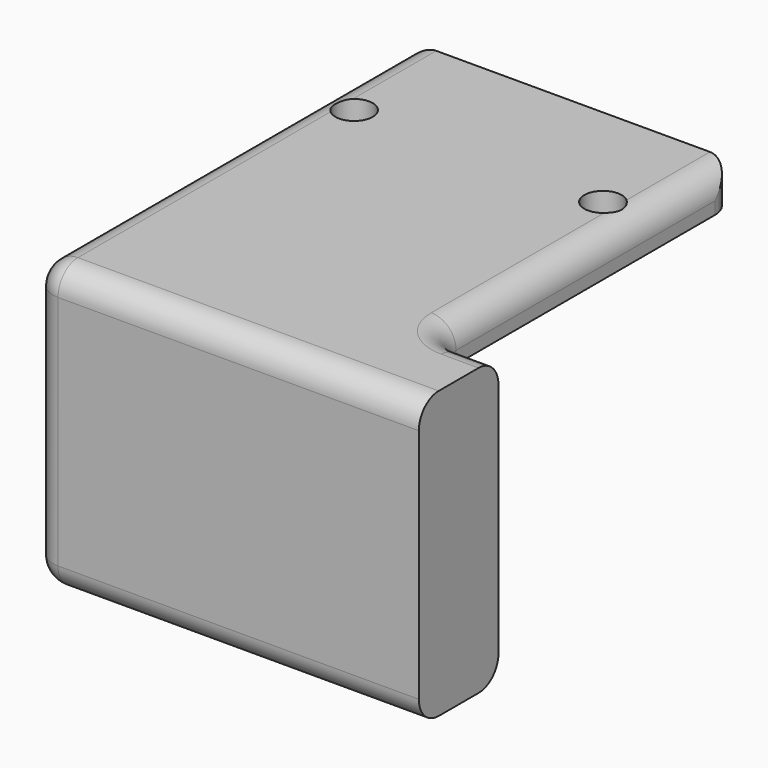
from build123d import *

# Parameters (mm, degrees)
F0_W         = 26
F0_H         = 38
F0_R         = 1.5
F1_DEPTH     = 3
F2_W         = 26
F2_H         = 8
F3_DEPTH     = 20
F5_DEPTH     = 5
F6_T1_DEPTH  = 3
F6_T3_DEPTH  = 18
F6_T5_DEPTH  = 19
F6_T7_DEPTH  = 13
F6_T9_DEPTH  = 41
F6_T11_DEPTH = 33
F6_T13_DEPTH = 34
F6_T15_DEPTH = 4
F6_T17_DEPTH = 8
F6_S21_W     = 2.04
F6_S21_H     = 2.04
F6_T22_DEPTH = 2.04
F6_S27_W     = 2.04
F6_S27_H     = 2.04
F6_T28_DEPTH = 2.04
F6_S33_W     = 2.04
F6_S33_H     = 2.04
F6_T34_DEPTH = 2.04
F6_T38_ANGLE = 90


# Not quite as in the source:
# - a fillet or chamfer that OpenCascade refuses, or shapes differently, is made with other operations: its cross-section is extruded or revolved along the edge and cut away or added


with BuildPart() as f1:
    # F0 (on Top) → F1 (new body)
    with BuildSketch(Plane.XY):
        Rectangle(F0_W, F0_H)
        with Locations((-10, 9.5)):
            Circle(F0_R, mode=Mode.SUBTRACT)
        with Locations((10, 9.5)):
            Circle(F0_R, mode=Mode.SUBTRACT)
    extrude(amount=F1_DEPTH)

    # F2 (on face) → F3 (join)
    with BuildSketch(Plane(origin=(0, 0, 0), x_dir=(1, 0, 0), z_dir=(0, 0, -1))):
        with Locations((0, 15)):
            Rectangle(F2_W, F2_H)
    extrude(amount=F3_DEPTH)

    # F4 (on face) → F5 (join)
    with BuildSketch(Plane.YZ.offset(13)):
        Polygon((-11, -20), (-11, 0), (-11, 3), (-19, 3), (-19, -20), align=None)
    extrude(amount=F5_DEPTH)

    # F6: fillet of radius 2 on 12 edges, made by hand

    # F6_s2 → F6_t1 (join)
    with BuildSketch(Plane.XY):
        with BuildLine():
            ThreePointArc((15, -11), (13.5857864376, -10.4142135624), (13, -9))
            Line((13, -9), (13, -11))
            Line((13, -11), (15, -11))
        make_face()
    extrude(amount=F6_T1_DEPTH)

    # F6_s4 → F6_t3 (cut)
    with BuildSketch(Plane.XY.offset(-18)):
        with BuildLine():
            ThreePointArc((-11, -11), (-12.4142135624, -11.5857864376), (-13, -13))
            Line((-13, -13), (-13, -11))
            Line((-13, -11), (-11, -11))
        make_face()
    extrude(amount=F6_T3_DEPTH, mode=Mode.SUBTRACT)

    # F6_s6 → F6_t5 (cut)
    with BuildSketch(Plane.XY.offset(-18)):
        with BuildLine():
            ThreePointArc((-11, -19), (-12.4142135624, -18.4142135624), (-13, -17))
            Line((-13, -17), (-13, -19))
            Line((-13, -19), (-11, -19))
        make_face()
    extrude(amount=F6_T5_DEPTH, mode=Mode.SUBTRACT)

    # F6_s8 → F6_t7 (cut)
    with BuildSketch(Plane.XY.offset(-5)):
        with BuildLine():
            ThreePointArc((13, 17), (12.4142135624, 18.4142135624), (11, 19))
            Line((11, 19), (13, 19))
            Line((13, 19), (13, 17))
        make_face()
        with BuildLine():
            ThreePointArc((-11, 19), (-12.4142135624, 18.4142135624), (-13, 17))
            Line((-13, 17), (-13, 19))
            Line((-13, 19), (-11, 19))
        make_face()
    extrude(amount=F6_T7_DEPTH, mode=Mode.SUBTRACT)

    # F6_s10 → F6_t9 (cut)
    with BuildSketch(Plane.XZ.offset(-24)):
        with BuildLine():
            ThreePointArc((-11, 3), (-12.4142135624, 2.4142135624), (-13, 1))
            Line((-13, 1), (-13, 3))
            Line((-13, 3), (-11, 3))
        make_face()
    extrude(amount=F6_T9_DEPTH, mode=Mode.SUBTRACT)

    # F6_s12 → F6_t11 (cut)
    with BuildSketch(Plane.XZ.offset(-24)):
        with BuildLine():
            ThreePointArc((13, 1), (12.4142135624, 2.4142135624), (11, 3))
            Line((11, 3), (13, 3))
            Line((13, 3), (13, 1))
        make_face()
    extrude(amount=F6_T11_DEPTH, mode=Mode.SUBTRACT)

    # F6_s14 → F6_t13 (cut)
    with BuildSketch(Plane.YZ.offset(-11)):
        with BuildLine():
            ThreePointArc((-13, -20), (-11.5857864376, -19.4142135624), (-11, -18))
            Line((-11, -18), (-11, -20))
            Line((-11, -20), (-13, -20))
        make_face()
        with BuildLine():
            ThreePointArc((-19, -18), (-18.4142135624, -19.4142135624), (-17, -20))
            Line((-17, -20), (-19, -20))
            Line((-19, -20), (-19, -18))
        make_face()
        with BuildLine():
            ThreePointArc((-19, 1), (-18.4142135624, 2.4142135624), (-17, 3))
            Line((-17, 3), (-19, 3))
            Line((-19, 3), (-19, 1))
        make_face()
    extrude(amount=F6_T13_DEPTH, mode=Mode.SUBTRACT)

    # F6_s16 → F6_t15 (cut)
    with BuildSketch(Plane.XZ.offset(13)):
        with BuildLine():
            ThreePointArc((-11, -20), (-12.4142135624, -19.4142135624), (-13, -18))
            Line((-13, -18), (-13, -20))
            Line((-13, -20), (-11, -20))
        make_face()
    extrude(amount=F6_T15_DEPTH, mode=Mode.SUBTRACT)

    # F6_s18 → F6_t17 (cut)
    with BuildSketch(Plane.YZ.offset(15)):
        with BuildLine():
            ThreePointArc((-11, 1), (-11.5857864376, 2.4142135624), (-13, 3))
            Line((-13, 3), (-11, 3))
            Line((-11, 3), (-11, 1))
        make_face()
    extrude(amount=F6_T17_DEPTH, mode=Mode.SUBTRACT)


with BuildPart() as f6_tool20:
    # F6_s21 → F6_t22 (new body)
    with BuildSketch(Plane.XY.offset(-18)):
        with Locations((-12.02, -11.98)):
            Rectangle(F6_S21_W, F6_S21_H)
    extrude(amount=-F6_T22_DEPTH)

    # F6_s23 → F6_t24 (revolve, cut)
    with BuildSketch(Plane(origin=(-11, -13, -18), x_dir=(0.7071067812, -0.7071067812, 0), z_dir=(0.7071067812, 0.7071067812, 0))):
        with BuildLine():
            ThreePointArc((0, -2), (2, 0), (0, 2))
            Line((0, 2), (0, -2))
        make_face()
    revolve(axis=Axis((-11, -13, -18), (0, 0, -1)), mode=Mode.SUBTRACT)


with BuildPart() as f1_1:
    add(f1.part)

    # F6_t19: cut F6_tool20
    add(f6_tool20.part, mode=Mode.SUBTRACT)


with BuildPart() as f6_tool26:
    # F6_s27 → F6_t28 (new body)
    with BuildSketch(Plane.XZ.offset(17)):
        with Locations((-12.02, 2.02)):
            Rectangle(F6_S27_W, F6_S27_H)
    extrude(amount=F6_T28_DEPTH)

    # F6_s29 → F6_t30 (revolve, cut)
    with BuildSketch(Plane(origin=(-11, -17, 1), x_dir=(0.7071067812, 0, -0.7071067812), z_dir=(-0.7071067812, 0, -0.7071067812))):
        with BuildLine():
            ThreePointArc((0, -2), (2, 0), (0, 2))
            Line((0, 2), (0, -2))
        make_face()
    revolve(axis=Axis((-11, -17, 1), (0, -1, 0)), mode=Mode.SUBTRACT)


with BuildPart() as f1_2:
    add(f1_1.part)

    # F6_t25: cut F6_tool26
    add(f6_tool26.part, mode=Mode.SUBTRACT)


with BuildPart() as f6_tool32:
    # F6_s33 → F6_t34 (new body)
    with BuildSketch(Plane.XZ.offset(17)):
        with Locations((-12.02, -19.02)):
            Rectangle(F6_S33_W, F6_S33_H)
    extrude(amount=F6_T34_DEPTH)

    # F6_s35 → F6_t36 (revolve, cut)
    with BuildSketch(Plane(origin=(-11, -17, -18), x_dir=(0.7071067812, 0, 0.7071067812), z_dir=(0.7071067812, 0, -0.7071067812))):
        with BuildLine():
            ThreePointArc((0, -2), (2, 0), (0, 2))
            Line((0, 2), (0, -2))
        make_face()
    revolve(axis=Axis((-11, -17, -18), (0, -1, 0)), mode=Mode.SUBTRACT)


with BuildPart() as f1_3:
    add(f1_2.part)

    # F6_t31: cut F6_tool32
    add(f6_tool32.part, mode=Mode.SUBTRACT)

    # F6_s37 → F6_t38 (revolve, cut)
    with BuildSketch(Plane.YZ.offset(15)):
        with BuildLine():
            ThreePointArc((-11, 1), (-11.5857864376, 2.4142135624), (-13, 3))
            Line((-13, 3), (-11, 3))
            Line((-11, 3), (-11, 1))
        make_face()
    revolve(axis=Axis((15, -9, 3), (0, 0, -1)), revolution_arc=F6_T38_ANGLE, mode=Mode.SUBTRACT)


solid = f1_3.part
